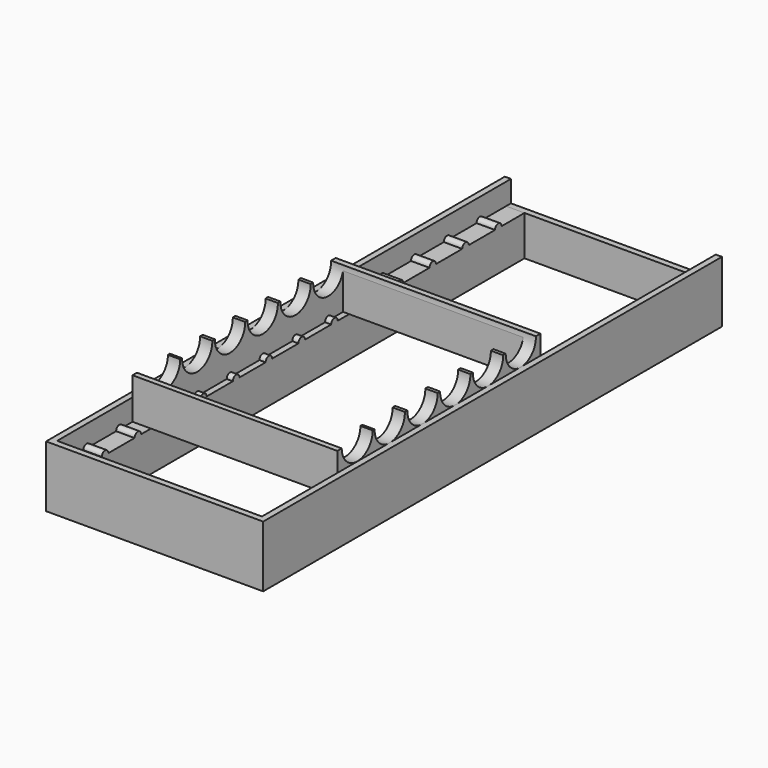
from build123d import *

# Parameters (mm, degrees)
F0_W      = 106
F0_H      = 280
F1_DEPTH  = 15
F2_W      = 82
F2_H      = 274
F3_DEPTH  = 39
F6_DEPTH  = 9
F7_DEPTH  = 9
F9_DEPTH  = 25
F11_DEPTH = 100
F12_W     = 88.0000000032
F12_H     = 111
F13_DEPTH = 25


# Not quite as in the source:
# - ends of sketch curves that miss each other by under 0.0002 mm in the source are joined


with BuildPart() as f1:
    # F0 (on Top) → F1 (new body, symmetric)
    with BuildSketch(Plane.XY):
        Rectangle(F0_W, F0_H)
    extrude(amount=F1_DEPTH, both=True)

    # F2 (on face) → F3 (cut)
    with BuildSketch(Plane.XY.offset(15)):
        Rectangle(F2_W, F2_H)
    extrude(amount=-F3_DEPTH, mode=Mode.SUBTRACT)

    # F4 (on face) → F6 (cut)
    with BuildSketch(Plane.YZ.offset(-41)):
        with BuildLine():
            Line((137, 15), (-137, 15))
            Line((-137, 15), (-137, 4.5))
            Line((-137, 4.5), (-121, 4.5))
            ThreePointArc((-121, 4.5), (-119, 6.5), (-117, 4.5))
            Line((-117, 4.5), (-101, 4.4999998063))
            ThreePointArc((-101, 4.4999998063), (-99, 6.4999998063), (-97, 4.4999998063))
            Line((-97, 4.4999998063), (-81, 4.4999998063))
            ThreePointArc((-81, 4.4999998063), (-79, 6.4999998063), (-77, 4.4999998063))
            Line((-77, 4.4999998063), (-61, 4.4999996126))
            ThreePointArc((-61, 4.4999996126), (-59, 6.4999996126), (-57, 4.4999996126))
            Line((-57, 4.4999996126), (-41.0000000298, 4.5))
            ThreePointArc((-41.0000000298, 4.5), (-39.0000000298, 6.5), (-37.0000000298, 4.5))
            Line((-37.0000000298, 4.5), (-21.0000000298, 4.4999998063))
            ThreePointArc((-21.0000000298, 4.4999998063), (-19.0000000298, 6.4999998063), (-17.0000000298, 4.4999998063))
            Line((-17.0000000298, 4.4999998063), (-1.0000000298, 4.4999998063))
            ThreePointArc((-1.0000000298, 4.4999998063), (0.9999999702, 6.4999998063), (2.9999999702, 4.4999998063))
            Line((2.9999999702, 4.4999998063), (18.9999999702, 4.4999996126))
            ThreePointArc((18.9999999702, 4.4999996126), (20.9999999702, 6.4999996126), (22.9999999702, 4.4999996126))
            Line((22.9999999702, 4.4999996126), (38.9999999702, 4.4999998063))
            ThreePointArc((38.9999999702, 4.4999998063), (40.9999999702, 6.4999998063), (42.9999999702, 4.4999998063))
            Line((42.9999999702, 4.4999998063), (58.9999999702, 4.4999996126))
            ThreePointArc((58.9999999702, 4.4999996126), (60.9999999702, 6.4999996126), (62.9999999702, 4.4999996126))
            Line((62.9999999702, 4.4999996126), (78.9999999702, 4.4999996126))
            ThreePointArc((78.9999999702, 4.4999996126), (80.9999999702, 6.4999996126), (82.9999999702, 4.4999996126))
            Line((82.9999999702, 4.4999996126), (98.9999999702, 4.4999994189))
            ThreePointArc((98.9999999702, 4.4999994189), (100.9999999702, 6.4999994189), (102.9999999702, 4.4999994189))
            Line((102.9999999702, 4.4999994189), (118.9999999404, 4.4999998063))
            ThreePointArc((118.9999999404, 4.4999998063), (120.9999999404, 6.4999998063), (122.9999999404, 4.4999998063))
            Line((122.9999999404, 4.4999998063), (137, 4.5))
            Line((137, 4.5), (137, 15))
        make_face()
    extrude(amount=-F6_DEPTH, mode=Mode.SUBTRACT)

    # F5 (on face) → F7 (cut)
    with BuildSketch(Plane(origin=(41, 0, 0), x_dir=(0, -1, 0), z_dir=(-1, 0, 0))):
        with BuildLine():
            Line((137, 4.5002960662), (137, 15))
            Line((137, 15), (-137, 15))
            Line((-137, 15), (-137, 4.5002960662))
            Line((-137, 4.5002960662), (-121, 4.5002960662))
            ThreePointArc((-121, 4.5002960662), (-119, 6.5002960662), (-117, 4.5002960662))
            Line((-117, 4.5002960662), (-101, 4.5002958725))
            ThreePointArc((-101, 4.5002958725), (-99, 6.5002958725), (-97, 4.5002958725))
            Line((-97, 4.5002958725), (-81, 4.5002958725))
            ThreePointArc((-81, 4.5002958725), (-79, 6.5002958725), (-77, 4.5002958725))
            Line((-77, 4.5002958725), (-61, 4.5002956788))
            ThreePointArc((-61, 4.5002956788), (-59, 6.5002956788), (-57, 4.5002956788))
            Line((-57, 4.5002956788), (-41.0000000298, 4.5002960662))
            ThreePointArc((-41.0000000298, 4.5002960662), (-39.0000000298, 6.5002960662), (-37.0000000298, 4.5002960662))
            Line((-37.0000000298, 4.5002960662), (-21.0000000298, 4.5002958725))
            ThreePointArc((-21.0000000298, 4.5002958725), (-19.0000000298, 6.5002958725), (-17.0000000298, 4.5002958725))
            Line((-17.0000000298, 4.5002958725), (-1.0000000298, 4.5002958725))
            ThreePointArc((-1.0000000298, 4.5002958725), (0.9999999702, 6.5002958725), (2.9999999702, 4.5002958725))
            Line((2.9999999702, 4.5002958725), (18.9999999702, 4.5002956788))
            ThreePointArc((18.9999999702, 4.5002956788), (20.9999999702, 6.5002956788), (22.9999999702, 4.5002956788))
            Line((22.9999999702, 4.5002956788), (38.9999999702, 4.5002958725))
            ThreePointArc((38.9999999702, 4.5002958725), (40.9999999702, 6.5002958725), (42.9999999702, 4.5002958725))
            Line((42.9999999702, 4.5002958725), (58.9999999702, 4.5002956788))
            ThreePointArc((58.9999999702, 4.5002956788), (60.9999999702, 6.5002956788), (62.9999999702, 4.5002956788))
            Line((62.9999999702, 4.5002956788), (78.9999999702, 4.5002956788))
            ThreePointArc((78.9999999702, 4.5002956788), (80.9999999702, 6.5002956788), (82.9999999702, 4.5002956788))
            Line((82.9999999702, 4.5002956788), (98.9999999702, 4.5002954851))
            ThreePointArc((98.9999999702, 4.5002954851), (100.9999999702, 6.5002954851), (102.9999999702, 4.5002954851))
            Line((102.9999999702, 4.5002954851), (118.9999999404, 4.5002958725))
            ThreePointArc((118.9999999404, 4.5002958725), (120.9999999404, 6.5002958725), (122.9999999404, 4.5002958725))
            Line((122.9999999404, 4.5002958725), (137, 4.5002960662))
        make_face()
    extrude(amount=-F7_DEPTH, mode=Mode.SUBTRACT)

    # F8 (on face) → F9 (cut)
    with BuildSketch(Plane.XZ.offset(-137)):
        Polygon((50, 15), (-50, 15), (-50, 4.5), (50, 4.5002960662), align=None)
    extrude(amount=-F9_DEPTH, mode=Mode.SUBTRACT)


with BuildPart() as f11:
    # F10 (on face) → F11 (new body, through all)
    with BuildSketch(Plane.YZ.offset(-50)):
        with BuildLine():
            ThreePointArc((-81, 4.4999998063), (-79, 6.4892055712), (-77, 4.4999998063))
            Line((-77, 4.4999998063), (-61, 4.4999996126))
            ThreePointArc((-61, 4.4999996126), (-59, 6.462326405), (-57, 4.4999996126))
            Line((-57, 4.4999996126), (-41.0000000298, 4.5))
            ThreePointArc((-41.0000000298, 4.5), (-39.0000000298, 6.5352561957), (-37.0000000298, 4.5))
            Line((-37.0000000298, 4.5), (-21.0000000298, 4.4999998063))
            ThreePointArc((-21.0000000298, 4.4999998063), (-19.0000000298, 6.4660892193), (-17.0000000298, 4.4999998063))
            Line((-17.0000000298, 4.4999998063), (-1.0000000298, 4.4999998063))
            ThreePointArc((-1.0000000298, 4.4999998063), (0.9999999702, 6.5320125012), (2.9999999702, 4.4999998063))
            Line((2.9999999702, 4.4999998063), (18.9999999702, 4.4999996126))
            ThreePointArc((18.9999999702, 4.4999996126), (20.9999999702, 6.5130431925), (22.9999999702, 4.4999996126))
            Line((22.9999999702, 4.4999996126), (32.9999999702, 4.4999998063))
            Line((32.9999999702, 4.4999998063), (32.9999999702, 24.4999998063))
            Line((32.9999999702, 24.4999998063), (31.7999999702, 24.4999998063))
            Line((31.7999999702, 24.4999998063), (30.1999999702, 24.4999998063))
            ThreePointArc((30.1999999702, 24.4999998063), (20.9999999702, 14.9057793253), (11.7999999702, 24.4999998063))
            Line((11.7999999702, 24.4999998063), (10.1999999702, 24.4999998063))
            ThreePointArc((10.1999999702, 24.4999998063), (0.9999999702, 14.9057793253), (-8.2000000298, 24.4999998063))
            Line((-8.2000000298, 24.4999998063), (-9.8000000298, 24.4999998063))
            ThreePointArc((-9.8000000298, 24.4999998063), (-19.0000000298, 14.9057793253), (-28.2000000298, 24.4999998063))
            Line((-28.2000000298, 24.4999998063), (-29.8000000298, 24.4999998063))
            ThreePointArc((-29.8000000298, 24.4999998063), (-39.0000000298, 14.9057793253), (-48.2000000298, 24.4999998063))
            Line((-48.2000000298, 24.4999998063), (-49.8, 24.4999998063))
            ThreePointArc((-49.8, 24.4999998063), (-59, 14.9057793253), (-68.2, 24.4999998063))
            Line((-68.2, 24.4999998063), (-69.3892873049, 24.4999998063))
            ThreePointArc((-69.3892873049, 24.4999998063), (-78.8531196296, 15.0361674815), (-88.3169519544, 24.4999998063))
            Line((-88.3169519544, 24.4999998063), (-89.9169519544, 24.4999998063))
            Line((-89.9169519544, 24.4999998063), (-91, 24.4999998063))
            Line((-91, 24.4999998063), (-91, 4.4999998063))
            Line((-91, 4.4999998063), (-81, 4.4999998063))
        make_face()
    extrude(amount=F11_DEPTH)

    # F12 (on face) → F13 (cut)
    with BuildSketch(Plane(origin=(0, 0, 4.4999998063), x_dir=(1, 0, 0), z_dir=(0, 0, -1))):
        with Locations((1.7e-09, 25.5)):
            Rectangle(F12_W, F12_H)
        Polygon((-44, 88), (-44, 86), (-43.9999999999, 81), (44.0000000017, 81), (44.0000000017, 86), (44.0000000017, 88), align=None)
    extrude(amount=-F13_DEPTH, mode=Mode.SUBTRACT)


solid = Compound([f1.part, f11.part])
